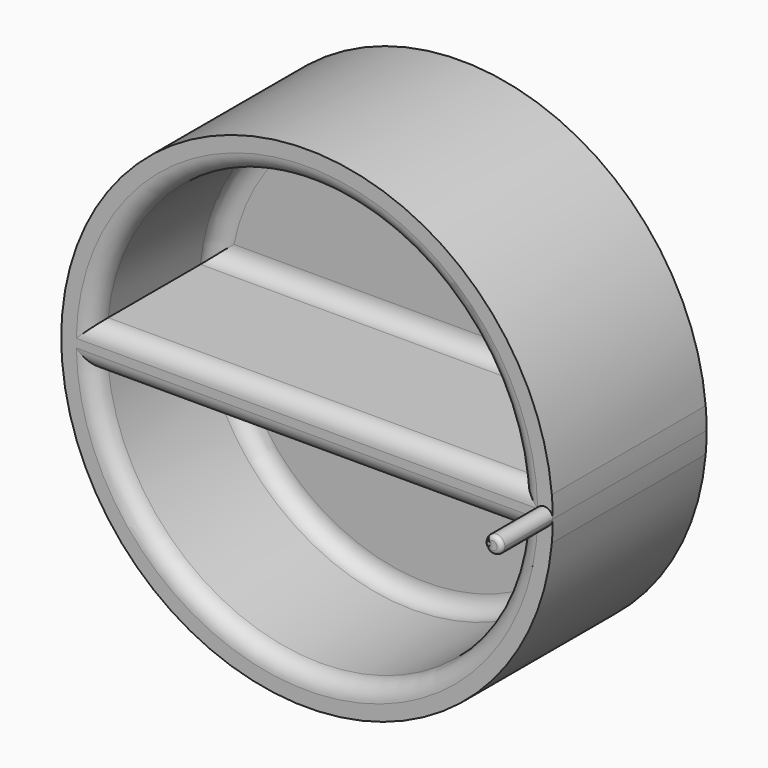
from build123d import *

# Parameters (mm, degrees)
F1_DEPTH     = 57.15
F2_DEPTH     = 12.7
F3_R         = 5.07999
F5_DEPTH     = 19.05
F6_T3_ANGLE  = 359.64
F6_T6_ANGLE  = 5.6286048719
F6_T10_ANGLE = 5.6286048719
F6_T14_DEPTH = 6.6329282975
F6_S15_R     = 68.5799900031
F6_T16_DEPTH = 5
F6_T19_ANGLE = 203.2655397093
F6_T22_DEPTH = 6.6329282975
F6_S23_R     = 68.5799900031
F6_T24_DEPTH = 5
F6_T27_ANGLE = 5.6286048719
F6_T31_ANGLE = 5.6286048719
F6_T36_ANGLE = 5.6286048719
F6_T41_DEPTH = 6.6329282975
F6_S42_R     = 68.5799900031
F6_T43_DEPTH = 5
F6_T48_DEPTH = 6.6329282975
F6_S49_R     = 68.5799900031
F6_T50_DEPTH = 5
F6_T53_ANGLE = 5.6286048719


# Not quite as in the source:
# - a fillet or chamfer that OpenCascade refuses, or shapes differently, is made with other operations: its cross-section is extruded or revolved along the edge and cut away or added
# - a fillet or chamfer is up to 0.001 mm smaller than in the source, because OpenCascade refuses the exact size


with BuildPart() as f1:
    # F0 (on Front) → F1 (new body)
    with BuildSketch(Plane.XZ):
        with BuildLine():
            ThreePointArc((72.7483891574, -6.35), (72.9558145154, -3.1780109172), (73.025, 0))
            ThreePointArc((73.025, 0), (72.9558145154, 3.1780109172), (72.7483891574, 6.35))
            Line((72.7483891574, 6.35), (63.1817022563, 6.35))
            ThreePointArc((63.1817022563, 6.35), (63.4203756425, 3.1789862163), (63.5, 0))
            ThreePointArc((63.5, 0), (63.4203756425, -3.1789862163), (63.1817022563, -6.35))
            Line((63.1817022563, -6.35), (72.7483891574, -6.35))
        make_face()
        with BuildLine():
            Line((63.1817022563, 6.35), (72.7483891574, 6.35))
            ThreePointArc((72.7483891574, 6.35), (0, 73.025), (-72.7483891574, 6.35))
            Line((-72.7483891574, 6.35), (-63.1817022563, 6.35))
            ThreePointArc((-63.1817022563, 6.35), (0, 63.5), (63.1817022563, 6.35))
        make_face()
        with BuildLine():
            ThreePointArc((-72.7483891574, -6.35), (0, -73.025), (72.7483891574, -6.35))
            Line((72.7483891574, -6.35), (63.1817022563, -6.35))
            ThreePointArc((63.1817022563, -6.35), (0, -63.5), (-63.1817022563, -6.35))
            Line((-63.1817022563, -6.35), (-72.7483891574, -6.35))
        make_face()
        with BuildLine():
            Line((-63.1817022563, 6.35), (-72.7483891574, 6.35))
            ThreePointArc((-72.7483891574, 6.35), (-73.025, 0), (-72.7483891574, -6.35))
            Line((-72.7483891574, -6.35), (-63.1817022563, -6.35))
            ThreePointArc((-63.1817022563, -6.35), (-63.5, 0), (-63.1817022563, 6.35))
        make_face()
        with BuildLine():
            ThreePointArc((63.5, 0), (63.4203756425, 3.1789862163), (63.1817022563, 6.35))
            Line((63.1817022563, 6.35), (-63.1817022563, 6.35))
            ThreePointArc((-63.1817022563, 6.35), (-63.5, 0), (-63.1817022563, -6.35))
            Line((-63.1817022563, -6.35), (63.1817022563, -6.35))
            ThreePointArc((63.1817022563, -6.35), (63.4203756425, -3.1789862163), (63.5, 0))
        make_face()
    extrude(amount=F1_DEPTH)

    # F0 (on Front) → F2 (join)
    with BuildSketch(Plane.XZ):
        with BuildLine():
            Line((-63.1817022563, 6.35), (63.1817022563, 6.35))
            ThreePointArc((63.1817022563, 6.35), (0, 63.5), (-63.1817022563, 6.35))
        make_face()
        with BuildLine():
            ThreePointArc((-63.1817022563, -6.35), (0, -63.5), (63.1817022563, -6.35))
            Line((63.1817022563, -6.35), (-63.1817022563, -6.35))
        make_face()
    extrude(amount=F2_DEPTH)

    # F3 (radius 5.08 in the source; OpenCascade refuses exactly that, so slightly less here)
    f3_edges = [f1.edges().sort_by_distance(p)[0] for p in [
        (0, -12.7, -6.35),
        (0, -12.7, -63.5),
        (0, -12.7, 63.5),
        (0, -12.7, 6.35),
        (0, -57.15, -63.5),
        (0, -57.15, 63.5),
        (0, -57.15, 6.35),
        (0, -57.15, -6.35),
    ]]
    fillet(f3_edges, radius=F3_R)

    # F4 (on face) → F5 (join)
    with BuildSketch(Plane.XZ.offset(57.15)):
        with BuildLine():
            ThreePointArc((68.5599677477, -1.6570609004), (71.3687471582, -2.3813002667), (73.025, 0))
            ThreePointArc((73.025, 0), (71.3687471582, 2.3813002667), (68.5599677477, 1.6570609004))
            ThreePointArc((68.5599677477, 1.6570609004), (68.5643717635, 1.46354128), (68.5682295455, 1.27001))
            Line((68.5682295455, 1.27001), (68.2853012479, 1.27001))
            ThreePointArc((68.2853012479, 1.27001), (67.945, 0), (68.2853012479, -1.27001))
            Line((68.2853012479, -1.27001), (68.5682295455, -1.27001))
            ThreePointArc((68.5682295455, -1.27001), (68.5643717635, -1.46354128), (68.5599677477, -1.6570609004))
        make_face()
    extrude(amount=F5_DEPTH)

    # F6: fillet of radius 1.27 on 6 edges, made by hand


with BuildPart() as f6_tool1:
    # F6_s2 → F6_t3 (revolve)
    with BuildSketch(Plane(origin=(0.0006956568, 0, 0.2214337012), x_dir=(0, 1, 0), z_dir=(-0.0031415875, 0, -0.9999950652))):
        with BuildLine():
            ThreePointArc((-74.93, 67.9446521708), (-75.8280256121, 68.3166265586), (-76.2, 69.2146521708))
            Line((-76.2, 69.2146521708), (-76.2, 67.9446521708))
            Line((-76.2, 67.9446521708), (-74.93, 67.9446521708))
        make_face()
    revolve(axis=Axis((70.485, -76.2, 0), (0, 1, 0)), revolution_arc=F6_T3_ANGLE)


with BuildPart() as f6_tool4:
    # F6_s5 → F6_t6 (revolve)
    with BuildSketch(Plane(origin=(0, 0, 2e-10), x_dir=(0, 1, 0), z_dir=(-0.0704028203, 0, 0.9975186429))):
        with BuildLine():
            ThreePointArc((-74.93, -68.57999), (-75.8280256121, -68.9519643879), (-76.2, -69.84999))
            Line((-76.2, -69.84999), (-76.2, -68.57999))
            Line((-76.2, -68.57999), (-74.93, -68.57999))
        make_face()
    revolve(axis=Axis((-3.1e-09, -76.2, -1e-10), (0, 1, 0)), revolution_arc=F6_T6_ANGLE)

    split(bisect_by=Plane.XY.offset(1.27001), keep=Keep.TOP)


with BuildPart() as f6_tool8:
    # F6_s9 → F6_t10 (revolve)
    with BuildSketch(Plane(origin=(0, 0, 2e-10), x_dir=(0, 1, 0), z_dir=(-0.0704028203, 0, 0.9975186429))):
        with BuildLine():
            ThreePointArc((-74.93, -68.57999), (-75.8280256121, -68.9519643879), (-76.2, -69.84999))
            Line((-76.2, -69.84999), (-76.2, -68.57999))
            Line((-76.2, -68.57999), (-74.93, -68.57999))
        make_face()
    revolve(axis=Axis((-3.1e-09, -76.2, -1e-10), (0, 1, 0)), revolution_arc=F6_T10_ANGLE)

    split(bisect_by=Plane.XY.offset(-1.27001), keep=Keep.BOTTOM)


with BuildPart() as f6_tool12:
    # F6_s13 → F6_t14 (new body)
    with BuildSketch(Plane.YZ.offset(71.7432295455)):
        with BuildLine():
            ThreePointArc((-74.93, 1.27001), (-75.8280256121, 0.8980356121), (-76.2, 1e-05))
            Line((-76.2, 1e-05), (-76.2, 1.27001))
            Line((-76.2, 1.27001), (-74.93, 1.27001))
        make_face()
    extrude(amount=-F6_T14_DEPTH)

    # F6_s15 → F6_t16 (intersect, symmetric)
    with BuildSketch(Plane.XZ.offset(75.6)):
        with Locations((-3.1e-09, -1e-10)):
            Circle(F6_S15_R)
    extrude(amount=F6_T16_DEPTH, both=True, mode=Mode.INTERSECT)


with BuildPart() as f6_tool17:
    # F6_s18 → F6_t19 (revolve)
    with BuildSketch(Plane(origin=(67.6192248978, 0, -13.9205420564), x_dir=(0, 1, 0), z_dir=(0.9794600845, 0, -0.2016381483))):
        with BuildLine():
            ThreePointArc((-74.93, 16.7524648841), (-75.8280256121, 16.3804904962), (-76.2, 15.4824648841))
            Line((-76.2, 15.4824648841), (-76.2, 16.7524648841))
            Line((-76.2, 16.7524648841), (-74.93, 16.7524648841))
        make_face()
    revolve(axis=Axis((70.485, -76.2, 0), (0, -1, 0)), revolution_arc=F6_T19_ANGLE)


with BuildPart() as f6_tool20:
    # F6_s21 → F6_t22 (new body)
    with BuildSketch(Plane.YZ.offset(65.1103012479)):
        with BuildLine():
            ThreePointArc((-76.2, -1e-05), (-75.8280256121, -0.8980356121), (-74.93, -1.27001))
            Line((-74.93, -1.27001), (-76.2, -1.27001))
            Line((-76.2, -1.27001), (-76.2, -1e-05))
        make_face()
    extrude(amount=F6_T22_DEPTH)

    # F6_s23 → F6_t24 (intersect, symmetric)
    with BuildSketch(Plane.XZ.offset(75.6)):
        with Locations((-3.1e-09, 1e-10)):
            Circle(F6_S23_R)
    extrude(amount=F6_T24_DEPTH, both=True, mode=Mode.INTERSECT)


with BuildPart() as f6_tool25:
    # F6_s26 → F6_t27 (revolve)
    with BuildSketch(Plane(origin=(0, 0, 2e-10), x_dir=(0, 1, 0), z_dir=(-0.027773006, 0, 0.9996142557))):
        with BuildLine():
            ThreePointArc((-76.2, -69.84999), (-75.8280256121, -68.9519643879), (-74.93, -68.57999))
            Line((-74.93, -68.57999), (-76.2, -68.57999))
            Line((-76.2, -68.57999), (-76.2, -69.84999))
        make_face()
    revolve(axis=Axis((-3.1e-09, -76.2, 1e-10), (0, 1, 0)), revolution_arc=F6_T27_ANGLE)

    split(bisect_by=Plane.XY.offset(1.27001), keep=Keep.TOP)


with BuildPart() as f6_tool29:
    # F6_s30 → F6_t31 (revolve)
    with BuildSketch(Plane(origin=(0, 0, 2e-10), x_dir=(0, 1, 0), z_dir=(-0.027773006, 0, 0.9996142557))):
        with BuildLine():
            ThreePointArc((-76.2, -69.84999), (-75.8280256121, -68.9519643879), (-74.93, -68.57999))
            Line((-74.93, -68.57999), (-76.2, -68.57999))
            Line((-76.2, -68.57999), (-76.2, -69.84999))
        make_face()
    revolve(axis=Axis((-3.1e-09, -76.2, 1e-10), (0, 1, 0)), revolution_arc=F6_T31_ANGLE)

    split(bisect_by=Plane.XY.offset(-1.27001), keep=Keep.BOTTOM)


with BuildPart() as f6_tool34:
    # F6_s35 → F6_t36 (revolve)
    with BuildSketch(Plane(origin=(0, 0, 2e-10), x_dir=(0, 1, 0), z_dir=(-0.0704028203, 0, 0.9975186429))):
        with BuildLine():
            ThreePointArc((-74.93, -68.57999), (-75.8280256121, -68.9519643879), (-76.2, -69.84999))
            Line((-76.2, -69.84999), (-76.2, -68.57999))
            Line((-76.2, -68.57999), (-74.93, -68.57999))
        make_face()
    revolve(axis=Axis((-3.1e-09, -76.2, -1e-10), (0, 1, 0)), revolution_arc=F6_T36_ANGLE)

    split(bisect_by=Plane.XY.offset(1.27001), keep=Keep.BOTTOM)

    split(bisect_by=Plane.XY.offset(-1.27001), keep=Keep.TOP)


with BuildPart() as f6_tool39:
    # F6_s40 → F6_t41 (new body)
    with BuildSketch(Plane.YZ.offset(71.7432295455)):
        with BuildLine():
            ThreePointArc((-74.93, 1.27001), (-75.8280256121, 0.8980356121), (-76.2, 1e-05))
            Line((-76.2, 1e-05), (-76.2, 1.27001))
            Line((-76.2, 1.27001), (-74.93, 1.27001))
        make_face()
    extrude(amount=-F6_T41_DEPTH)

    # F6_s42 → F6_t43 (cut, symmetric)
    with BuildSketch(Plane.XZ.offset(75.6)):
        with Locations((-3.1e-09, -1e-10)):
            Circle(F6_S42_R)
    extrude(amount=F6_T43_DEPTH, both=True, mode=Mode.SUBTRACT)


with BuildPart() as f6_tool34_1:
    add(f6_tool34.part)

    # F6_t44: intersect F6_tool39
    add(f6_tool39.part, mode=Mode.INTERSECT)


with BuildPart() as f6_tool46:
    # F6_s47 → F6_t48 (new body)
    with BuildSketch(Plane.YZ.offset(65.1103012479)):
        with BuildLine():
            ThreePointArc((-76.2, -1e-05), (-75.8280256121, -0.8980356121), (-74.93, -1.27001))
            Line((-74.93, -1.27001), (-76.2, -1.27001))
            Line((-76.2, -1.27001), (-76.2, -1e-05))
        make_face()
    extrude(amount=F6_T48_DEPTH)

    # F6_s49 → F6_t50 (cut, symmetric)
    with BuildSketch(Plane.XZ.offset(75.6)):
        with Locations((-3.1e-09, 1e-10)):
            Circle(F6_S49_R)
    extrude(amount=F6_T50_DEPTH, both=True, mode=Mode.SUBTRACT)


with BuildPart() as f6_tool51:
    # F6_s52 → F6_t53 (revolve)
    with BuildSketch(Plane(origin=(0, 0, 2e-10), x_dir=(0, 1, 0), z_dir=(-0.027773006, 0, 0.9996142557))):
        with BuildLine():
            ThreePointArc((-76.2, -69.84999), (-75.8280256121, -68.9519643879), (-74.93, -68.57999))
            Line((-74.93, -68.57999), (-76.2, -68.57999))
            Line((-76.2, -68.57999), (-76.2, -69.84999))
        make_face()
    revolve(axis=Axis((-3.1e-09, -76.2, 1e-10), (0, 1, 0)), revolution_arc=F6_T53_ANGLE)

    split(bisect_by=Plane.XY.offset(1.27001), keep=Keep.BOTTOM)

    split(bisect_by=Plane.XY.offset(-1.27001), keep=Keep.TOP)


with BuildPart() as f6_tool46_1:
    add(f6_tool46.part)

    # F6_t56: intersect F6_tool51
    add(f6_tool51.part, mode=Mode.INTERSECT)


with BuildPart() as f1_1:
    add(f1.part)

    # F6_t57: cut F6_tool1, F6_tool4, F6_tool8, F6_tool12, F6_tool17, F6_tool20, F6_tool25, F6_tool29, F6_tool34, F6_tool46
    add([f6_tool1.part, f6_tool4.part, f6_tool8.part, f6_tool12.part, f6_tool17.part, f6_tool20.part, f6_tool25.part, f6_tool29.part, f6_tool34_1.part, f6_tool46_1.part], mode=Mode.SUBTRACT)


solid = f1_1.part
